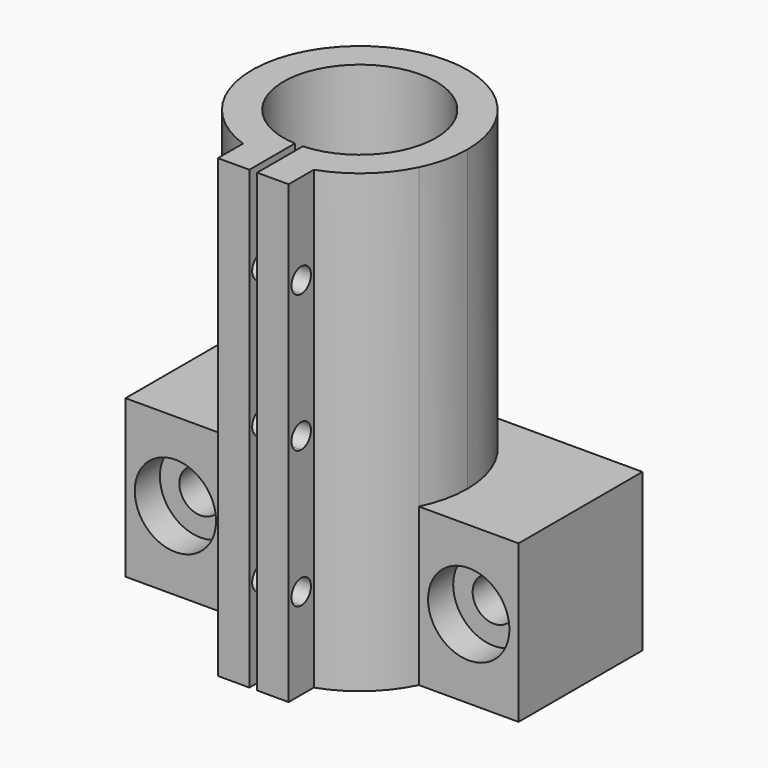
from build123d import *

# Parameters (mm, degrees)
F1_DEPTH = 20
F0_W     = 4
F0_H     = 2.9398608957
F2_DEPTH = 58
F4_DEPTH = 4
F5_DEPTH = 20
F7_DEPTH = 9


# Not quite as in the source:
# - a feature names something its author has since deleted; it is built from what else it names


with BuildPart() as f1:
    # F0 (on Top) → F1 (new body)
    with BuildSketch(Plane.XY):
        with BuildLine():
            Line((0, 13.7), (-25, 13.7))
            Line((-25, 13.7), (-25, -6))
            Line((-25, -6), (-12.3162494291, -6))
            ThreePointArc((-12.3162494291, -6), (-11.6165829744, 7.2625753008), (0, 13.7))
        make_face()
    extrude(amount=F1_DEPTH)



with BuildPart() as f1b:
    # F0 (on Top) → F1, piece 2 (new body)
    with BuildSketch(Plane.XY):
        with BuildLine():
            Line((25, 13.7), (0, 13.7))
            ThreePointArc((0, 13.7), (9.6873629023, 9.6873629023), (13.7, 0))
            ThreePointArc((13.7, 0), (13.3495808395, -3.0787483513), (12.3162494291, -6))
            Line((12.3162494291, -6), (25, -6))
            Line((25, -6), (25, 13.7))
        make_face()
    extrude(amount=F1_DEPTH)


with BuildPart() as f1_1:
    add(f1.part)

    add(f1b.part)  # F2 merges F1b
    # F0 (on Top) → F2 (join)
    with BuildSketch(Plane.XY):
        with BuildLine():
            ThreePointArc((13.7, 0), (9.6873629023, 9.6873629023), (0, 13.7))
            ThreePointArc((0, 13.7), (-11.6165829744, 7.2625753008), (-12.3162494291, -6))
            Line((-12.3162494291, -6), (-7.6216796049, -6))
            ThreePointArc((-7.6216796049, -6), (-3.1748785672, 9.1657048875), (9.7, 0))
            ThreePointArc((9.7, 0), (9.1657048875, -3.1748785672), (7.6216796049, -6))
            Line((7.6216796049, -6), (12.3162494291, -6))
            ThreePointArc((12.3162494291, -6), (13.3495808395, -3.0787483513), (13.7, 0))
        make_face()
        with BuildLine():
            Line((-7.6216796049, -6), (-12.3162494291, -6))
            ThreePointArc((-12.3162494291, -6), (-9.0959869464, -10.244658192), (-4.5, -12.9398608957))
            ThreePointArc((-4.5, -12.9398608957), (-2.5280436601, -13.4647315329), (-0.5, -13.6908728721))
            Line((-0.5, -13.6908728721), (-0.5, -9.6871048306))
            ThreePointArc((-0.5, -9.6871048306), (-4.4597203286, -8.6139941137), (-7.6216796049, -6))
        make_face()
        with BuildLine():
            ThreePointArc((4.5, -12.9398608957), (9.0959869464, -10.244658192), (12.3162494291, -6))
            Line((12.3162494291, -6), (7.6216796049, -6))
            ThreePointArc((7.6216796049, -6), (4.4597203286, -8.6139941137), (0.5, -9.6871048306))
            Line((0.5, -9.6871048306), (0.5, -13.6908728721))
            ThreePointArc((0.5, -13.6908728721), (2.5280436601, -13.4647315329), (4.5, -12.9398608957))
        make_face()
        with Locations((2.5, -15.4699304478)):
            Rectangle(F0_W, F0_H)
        with BuildLine():
            Line((4.5, -14), (4.5, -12.9398608957))
            ThreePointArc((4.5, -12.9398608957), (2.5280436601, -13.4647315329), (0.5, -13.6908728721))
            Line((0.5, -13.6908728721), (0.5, -14))
            Line((0.5, -14), (4.5, -14))
        make_face()
        with BuildLine():
            ThreePointArc((-0.5, -13.6908728721), (-2.5280436601, -13.4647315329), (-4.5, -12.9398608957))
            Line((-4.5, -12.9398608957), (-4.5, -14))
            Line((-4.5, -14), (-0.5, -14))
            Line((-0.5, -14), (-0.5, -13.6908728721))
        make_face()
        with Locations((-2.5, -15.4699304478)):
            Rectangle(F0_W, F0_H)
    extrude(amount=F2_DEPTH)

    # F3 (on face) → F4 (cut)
    with BuildSketch(Plane.XZ.offset(6)):
        with BuildLine():
            ThreePointArc((-21.3581247146, 10), (-18.6581247146, 12.7), (-15.9581247146, 10))
            Line((-15.9581247146, 10), (-13.4831247146, 10))
            ThreePointArc((-13.4831247146, 10), (-18.6581247146, 15.175), (-23.8331247146, 10))
            Line((-23.8331247146, 10), (-21.3581247146, 10))
        make_face()
        with BuildLine():
            Line((-13.4831247146, 10), (-15.9581247146, 10))
            ThreePointArc((-15.9581247146, 10), (-18.6581247146, 7.3), (-21.3581247146, 10))
            Line((-21.3581247146, 10), (-23.8331247146, 10))
            ThreePointArc((-23.8331247146, 10), (-18.6581247146, 4.825), (-13.4831247146, 10))
        make_face()
        with BuildLine():
            ThreePointArc((23.8331247146, 10), (18.6581247146, 15.175), (13.4831247146, 10))
            Line((13.4831247146, 10), (15.9581247146, 10))
            ThreePointArc((15.9581247146, 10), (18.6581247146, 12.7), (21.3581247146, 10))
            Line((21.3581247146, 10), (23.8331247146, 10))
        make_face()
        with BuildLine():
            Line((15.9581247146, 10), (13.4831247146, 10))
            ThreePointArc((13.4831247146, 10), (18.6581247146, 4.825), (23.8331247146, 10))
            Line((23.8331247146, 10), (21.3581247146, 10))
            ThreePointArc((21.3581247146, 10), (18.6581247146, 7.3), (15.9581247146, 10))
        make_face()
    extrude(amount=-F4_DEPTH, mode=Mode.SUBTRACT)

    # F5 (cut): faces of the model
    f5_faces = [f1_1.faces().sort_by_distance(p)[0] for p in [
        (-18.6581247146, -6, 10),
        (18.6581247146, -6, 10),
    ]]
    extrude(f5_faces, amount=-F5_DEPTH, mode=Mode.SUBTRACT)

    # F6 (on face) → F7 (cut)
    with BuildSketch(Plane(origin=(-4.5, 0, 0), x_dir=(0, -1, 0), z_dir=(-1, 0, 0))):
        with BuildLine():
            ThreePointArc((16.4898608957, 46.45), (16.0358764065, 47.5460155108), (14.9398608957, 48))
            Line((14.9398608957, 48), (14.9398608957, 44.9))
            ThreePointArc((14.9398608957, 44.9), (16.0358764065, 45.3539844892), (16.4898608957, 46.45))
        make_face()
        with BuildLine():
            ThreePointArc((16.4898608957, 11.55), (16.0358764065, 12.6460155108), (14.9398608957, 13.1))
            Line((14.9398608957, 13.1), (14.9398608957, 10))
            ThreePointArc((14.9398608957, 10), (16.0358764065, 10.4539844892), (16.4898608957, 11.55))
        make_face()
        with BuildLine():
            Line((14.9398608957, 10), (14.9398608957, 13.1))
            ThreePointArc((14.9398608957, 13.1), (13.3898608957, 11.55), (14.9398608957, 10))
        make_face()
        with BuildLine():
            ThreePointArc((16.4898608957, 29), (16.0358764065, 30.0960155108), (14.9398608957, 30.55))
            Line((14.9398608957, 30.55), (14.9398608957, 29))
            Line((14.9398608957, 29), (16.4898608957, 29))
        make_face()
        with BuildLine():
            Line((14.9398608957, 29), (14.9398608957, 30.55))
            ThreePointArc((14.9398608957, 30.55), (13.3898608957, 29), (14.9398608957, 27.45))
            Line((14.9398608957, 27.45), (14.9398608957, 29))
        make_face()
        with BuildLine():
            Line((14.9398608957, 44.9), (14.9398608957, 48))
            ThreePointArc((14.9398608957, 48), (13.3898608957, 46.45), (14.9398608957, 44.9))
        make_face()
        with BuildLine():
            Line((16.4898608957, 29), (14.9398608957, 29))
            Line((14.9398608957, 29), (14.9398608957, 27.45))
            ThreePointArc((14.9398608957, 27.45), (16.0358764065, 27.9039844892), (16.4898608957, 29))
        make_face()
    extrude(amount=-F7_DEPTH, mode=Mode.SUBTRACT)


solid = f1_1.part
